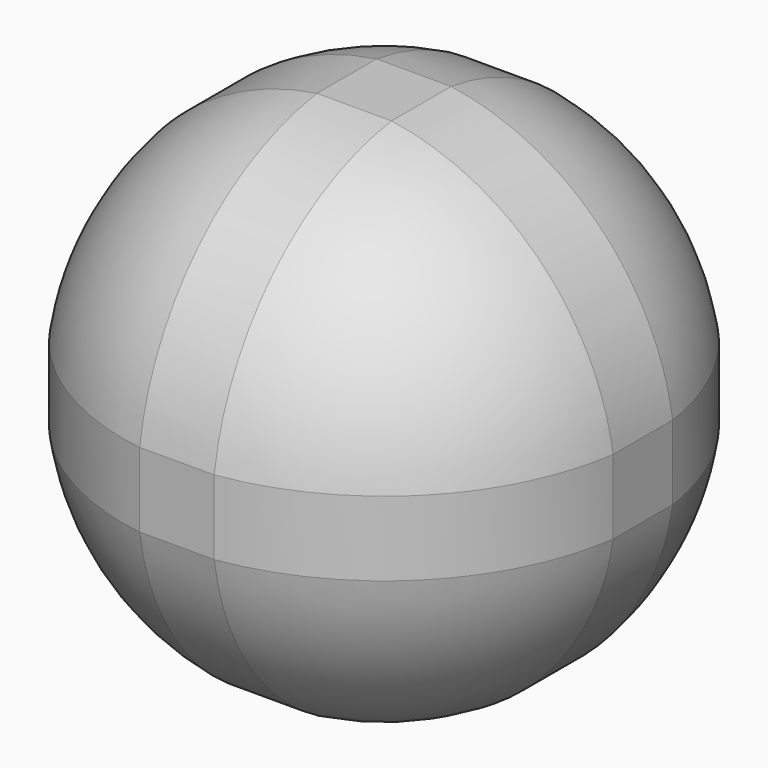
from build123d import *

# Parameters (mm, degrees)
F3_R           = 131.0263205289
F3_R_2         = 49.5
F4_DEPTH       = 110.001
F7_R           = 68.9137805215
F7_R_2         = 49.5
F8_DEPTH       = 109.5010000999
F9_R           = 79.7088891181
F9_R_2         = 49.5
F10_DEPTH      = 109.5010001
F17_W          = 10.0190378726
F17_H          = 14.1067359797
F17_W_2        = 14.1067359797
F17_H_2        = 10.022751987
F17_W_3        = 14.5319104195
F17_H_3        = 15.0359645486
F18_DEPTH      = 49.5010001
F18_DEPTH_BACK = 49.5010001
F19_W          = 14.1067359797
F19_H          = 7.9913586378
F20_DEPTH      = 48.9958977935
F20_DEPTH_BACK = 25


# Not quite as in the source:
# - a feature of the source that left no trace in its solid (it failed there, or was rolled back) is left out
# - a pattern or mirror of a feature is missing from the dataset's text; its kind, count and spacing are read off the source's solid


with BuildPart() as f1:
    # F0 (on Top) → F1 (revolve)
    with BuildSketch(Plane.XY):
        with BuildLine():
            Line((0, 0), (50, 0))
            ThreePointArc((50, 0), (0, 50), (-50, 0))
            Line((-50, 0), (0, 0))
        make_face()
    revolve(axis=Axis((6.9401971996, 0, 0), (1, 0, 0)))

    # F3 (on offset) → F4 (cut, through all)
    with BuildSketch(Plane.XY.offset(60)):
        Circle(F3_R)
        Circle(F3_R_2, mode=Mode.SUBTRACT)
    extrude(amount=-F4_DEPTH, mode=Mode.SUBTRACT)

    # F7 (on offset) → F8 (cut, through all)
    with BuildSketch(Plane.XZ.offset(60)):
        Circle(F7_R)
        Circle(F7_R_2, mode=Mode.SUBTRACT)
    extrude(amount=-F8_DEPTH, mode=Mode.SUBTRACT)

    # F9 (on offset) → F10 (cut, through all)
    with BuildSketch(Plane.YZ.offset(60)):
        Circle(F9_R)
        Circle(F9_R_2, mode=Mode.SUBTRACT)
    extrude(amount=-F10_DEPTH, mode=Mode.SUBTRACT)

    # F17 (on Top) → F18 (cut, two sides)
    with BuildSketch(Plane.XY) as f18_sk:
        with Locations((-54.0044166298, 0)):
            Rectangle(F17_W, F17_H)
        with Locations((0, 54.006273687)):
            Rectangle(F17_W_2, F17_H_2)
        with Locations((56.2608529033, 0)):
            Rectangle(F17_W_3, F17_H)
        with Locations((0, -56.5128799678)):
            Rectangle(F17_W_2, F17_H_3)
    extrude(amount=-F18_DEPTH, mode=Mode.SUBTRACT)
    extrude(f18_sk.sketch, amount=F18_DEPTH_BACK, mode=Mode.SUBTRACT)

    # F19 (on Front) → F20 (cut, two sides)
    with BuildSketch(Plane.XZ) as f20_sk:
        with Locations((0, -52.9905770124)):
            Rectangle(F19_W, F19_H)
    f20 = extrude(amount=-F20_DEPTH, mode=Mode.SUBTRACT) + extrude(f20_sk.sketch, amount=F20_DEPTH_BACK, mode=Mode.SUBTRACT)

    # F20_copies: F20 across plane
    add(f20.mirror(Plane.XY), mode=Mode.SUBTRACT)


solid = f1.part
